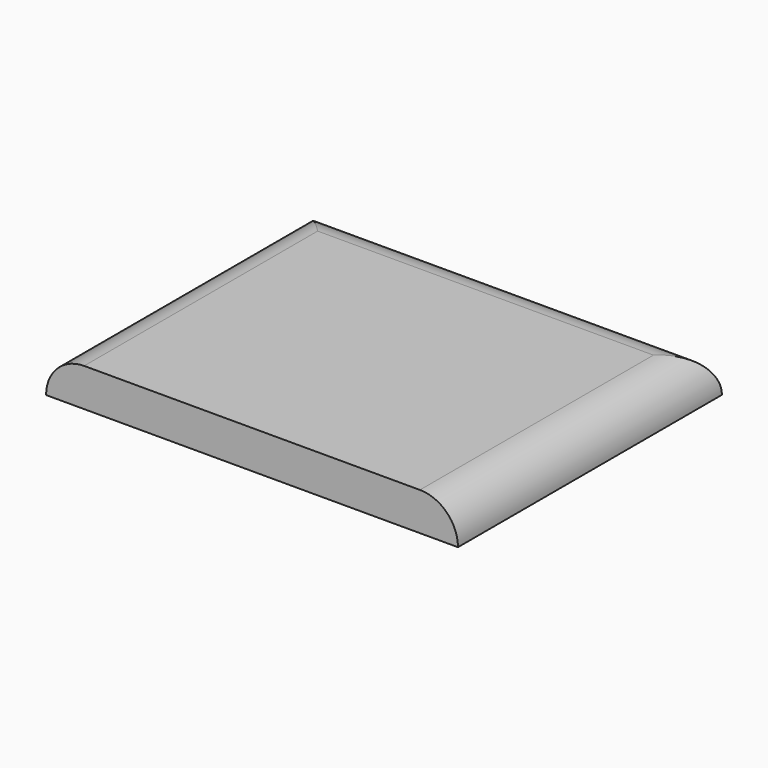
from build123d import *

# Parameters (mm, degrees)
F0_W     = 68.736359477
F0_H     = 55.0630092621
F1_DEPTH = 6.35
F2_R     = 6.34999


# Not quite as in the source:
# - a fillet or chamfer is up to 0.001 mm smaller than in the source, because OpenCascade refuses the exact size


with BuildPart() as f1:
    # F0 (on Top) → F1 (new body)
    with BuildSketch(Plane.XY):
        with Locations((-7.4506e-06, 2.0325183868)):
            Rectangle(F0_W, F0_H)
    extrude(amount=F1_DEPTH)

    # F2 (radius 6.35 in the source; OpenCascade refuses exactly that, so slightly less here)
    f2_edges = [f1.edges().sort_by_distance(p)[0] for p in [
        (-7e-06, 29.564023, 6.35),
        (34.368172, 2.032518, 6.35),
        (-34.368187, 2.032518, 6.35),
    ]]
    fillet(f2_edges, radius=F2_R)


solid = f1.part
